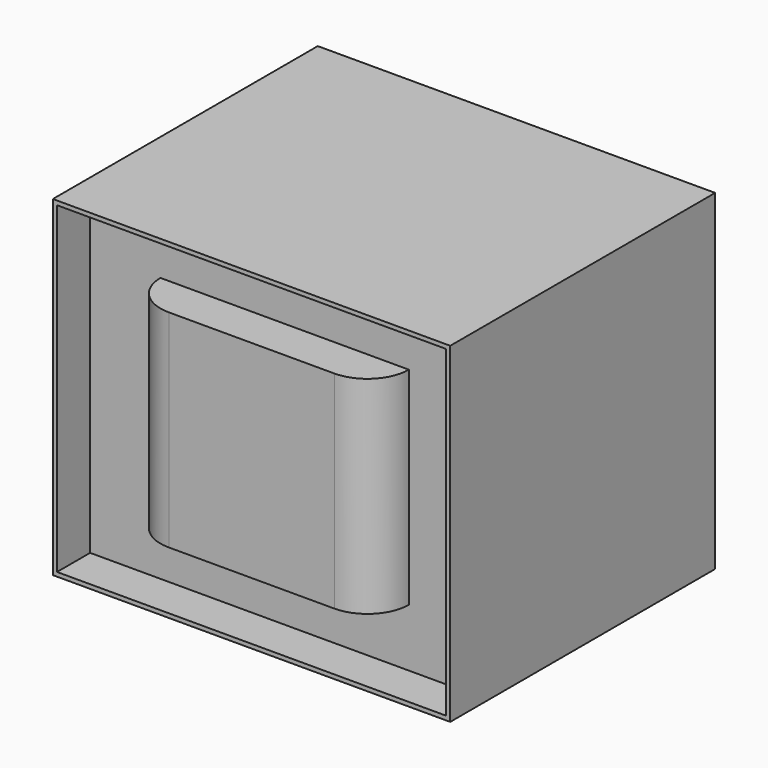
from build123d import *

# Parameters (mm, degrees)
F0_W     = 96
F0_H     = 80
F1_DEPTH = 80
F2_W     = 94
F2_H     = 78
F2_W_2   = 60
F2_H_2   = 50
F3_DEPTH = 10
F4_R     = 9.99999


# Not quite as in the source:
# - a fillet or chamfer is up to 0.001 mm smaller than in the source, because OpenCascade refuses the exact size
# - a pattern or mirror of a feature is missing from the dataset's text; its kind, count and spacing are read off the source's solid


with BuildPart() as f1:
    # F0 (on Top) → F1 (new body)
    with BuildSketch(Plane.XY):
        Rectangle(F0_W, F0_H)
    extrude(amount=F1_DEPTH)

    # F2 (on face) → F3 (cut)
    with BuildSketch(Plane.XZ.offset(40)):
        with Locations((0, 40)):
            Rectangle(F2_W, F2_H)
        with Locations((0, 40)):
            Rectangle(F2_W_2, F2_H_2, mode=Mode.SUBTRACT)
    f3 = extrude(amount=-F3_DEPTH, mode=Mode.SUBTRACT)

    # F3_copies: F3 across plane
    add(f3.mirror(Plane.ZX), mode=Mode.SUBTRACT)

    # F4 (radius 10 in the source; OpenCascade refuses exactly that, so slightly less here)
    f4_edges = [f1.edges().sort_by_distance(p)[0] for p in [
        (30, -40, 40),
        (-30, -40, 40),
        (30, 40, 40),
        (-30, 40, 40),
    ]]
    fillet(f4_edges, radius=F4_R)


solid = f1.part
